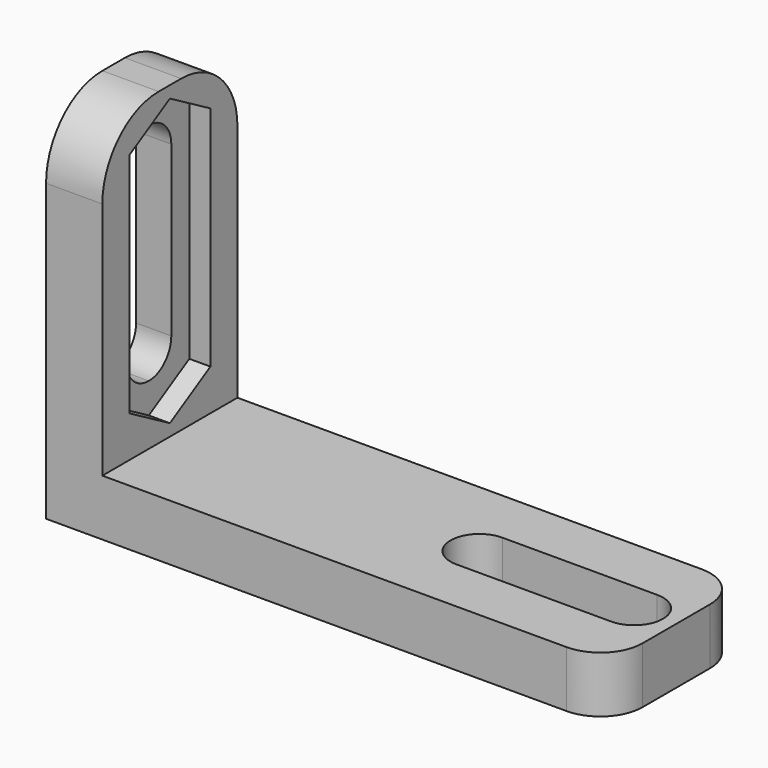
from build123d import *

# Parameters (mm, degrees)
F1_DEPTH = 4
F2_W     = 4
F2_H     = 12
F3_DEPTH = 22
F5_DEPTH = 25
F7_DEPTH = 1.5
F8_R     = 5


# Not quite as in the source:
# - a feature names something its author has since deleted; it is built from what else it names


with BuildPart() as f1:
    # F0 (on Top) → F1 (new body)
    with BuildSketch(Plane.XY):
        with BuildLine():
            ThreePointArc((0, -3), (-0.8786796564, -0.8786796564), (-3, 0))
            Line((-3, 0), (-40, 0))
            Line((-40, 0), (-40, -12))
            Line((-40, -12), (-3, -12))
            ThreePointArc((-3, -12), (-0.8786796564, -11.1213203436), (0, -9))
            Line((0, -9), (0, -3))
        make_face()
        with BuildLine():
            ThreePointArc((-3, -3.95), (-0.95, -6), (-3, -8.05))
            Line((-3, -8.05), (-14, -8.05))
            ThreePointArc((-14, -8.05), (-16.05, -6), (-14, -3.95))
            Line((-14, -3.95), (-3, -3.95))
        make_face(mode=Mode.SUBTRACT)
    extrude(amount=F1_DEPTH)

    # F2 (on face) → F3 (join)
    with BuildSketch(Plane.XY.offset(4)):
        with Locations((-38, -6)):
            Rectangle(F2_W, F2_H)
    extrude(amount=F3_DEPTH)

    # F4 (on face) → F5 (cut)
    with BuildSketch(Plane(origin=(-40, 0, 0), x_dir=(0, -1, 0), z_dir=(-1, 0, 0))):
        with BuildLine():
            Line((4, 21), (4, 9))
            ThreePointArc((4, 9), (4.5857864376, 7.5857864376), (6, 7))
            ThreePointArc((6, 7), (7.4142135624, 7.5857864376), (8, 9))
            Line((8, 9), (8, 21))
            ThreePointArc((8, 21), (7.4142135624, 22.4142135624), (6, 23))
            ThreePointArc((6, 23), (4.5857864376, 22.4142135624), (4, 21))
        make_face()
    extrude(amount=-F5_DEPTH, mode=Mode.SUBTRACT)

    # F6 (on face) → F7 (cut)
    with BuildSketch(Plane.YZ.offset(-36)):
        Polygon((-6, 4.8430780618), (-2.4, 6.9215390309), (-2.4, 23.0784609691), (-6, 25.1569219382), (-9.6, 23.0784609691), (-9.6, 6.9215390309), align=None)
        with BuildLine():
            ThreePointArc((-8, 21), (-6, 23), (-4, 21))
            Line((-4, 21), (-4, 9))
            ThreePointArc((-4, 9), (-6, 7), (-8, 9))
            Line((-8, 9), (-8, 21))
        make_face(mode=Mode.SUBTRACT)
    extrude(amount=-F7_DEPTH, mode=Mode.SUBTRACT)

    # F8
    f8_edges = [f1.edges().sort_by_distance(p)[0] for p in [
        (-38, -12, 26),
        (-38, 0, 26),
    ]]
    fillet(f8_edges, radius=F8_R)


solid = f1.part
